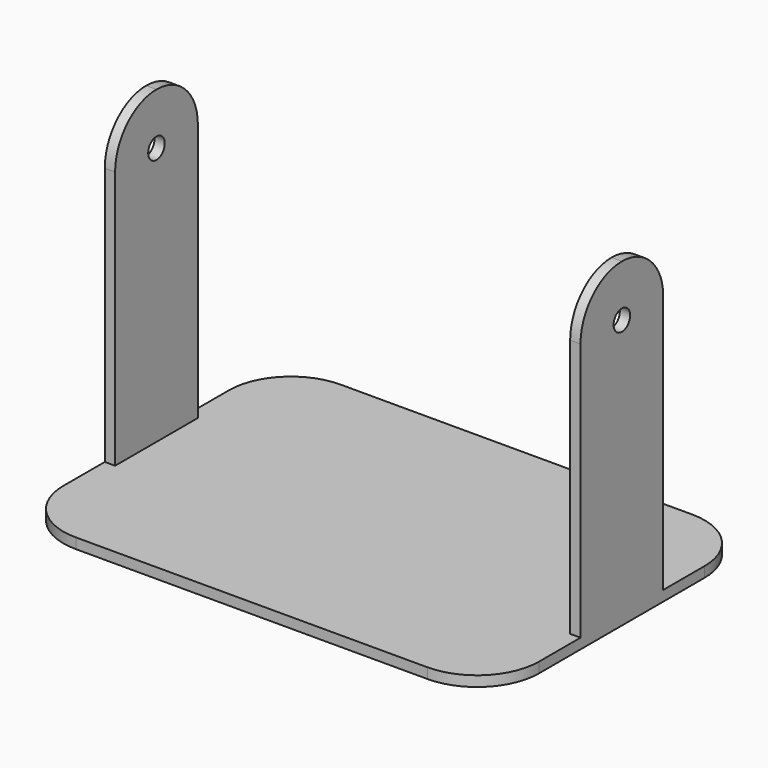
from build123d import *

# Parameters (mm, degrees)
F1_DEPTH = 50
F2_R     = 24.99999
F3_R     = 5
F4_DEPTH = 230.001
F6_DEPTH = 5


# Not quite as in the source:
# - a fillet or chamfer is up to 0.001 mm smaller than in the source, because OpenCascade refuses the exact size


with BuildPart() as f1:
    # F0 (on Front) → F1 (new body)
    with BuildSketch(Plane.XZ):
        Polygon((-119.9185385572, 72.4322550792), (-119.9185385572, -82.5677449208), (110.0814614428, -82.5677449208), (110.0814614428, 72.4322550792), (105.0814614428, 72.4322550792), (105.0814614428, -77.5677449208), (-114.9185385572, -77.5677449208), (-114.9185385572, 72.4322550792), align=None)
    extrude(amount=F1_DEPTH)

    # F2 (radius 25 in the source; OpenCascade refuses exactly that, so slightly less here)
    f2_edges = [f1.edges().sort_by_distance(p)[0] for p in [
        (-117.418539, -50, 72.432255),
        (-117.418539, 0, 72.432255),
        (107.581461, -50, 72.432255),
        (107.581461, 0, 72.432255),
    ]]
    fillet(f2_edges, radius=F2_R)

    # F3 (on face) → F4 (cut, through all)
    with BuildSketch(Plane(origin=(-119.9185385572, 0, 0), x_dir=(0, -1, 0), z_dir=(-1, 0, 0))):
        with Locations((25, 47.4322550792)):
            Circle(F3_R)
    extrude(amount=-F4_DEPTH, mode=Mode.SUBTRACT)

    # F5 (on face) → F6 (join)
    with BuildSketch(Plane(origin=(0, 0, -82.5677449208), x_dir=(1, 0, 0), z_dir=(0, 0, -1))):
        with BuildLine():
            Line((80.0814614428, 105), (-89.9185385572, 105))
            ThreePointArc((-89.9185385572, 105), (-111.1317419928, 96.2132034356), (-119.9185385572, 75))
            Line((-119.9185385572, 75), (-119.9185385572, -25))
            ThreePointArc((-119.9185385572, -25), (-111.1317419928, -46.2132034356), (-89.9185385572, -55))
            Line((-89.9185385572, -55), (80.0814614428, -55))
            ThreePointArc((80.0814614428, -55), (101.2946648784, -46.2132034356), (110.0814614428, -25))
            Line((110.0814614428, -25), (110.0814614428, 75))
            ThreePointArc((110.0814614428, 75), (101.2946648784, 96.2132034356), (80.0814614428, 105))
        make_face()
    extrude(amount=-F6_DEPTH)


solid = f1.part
